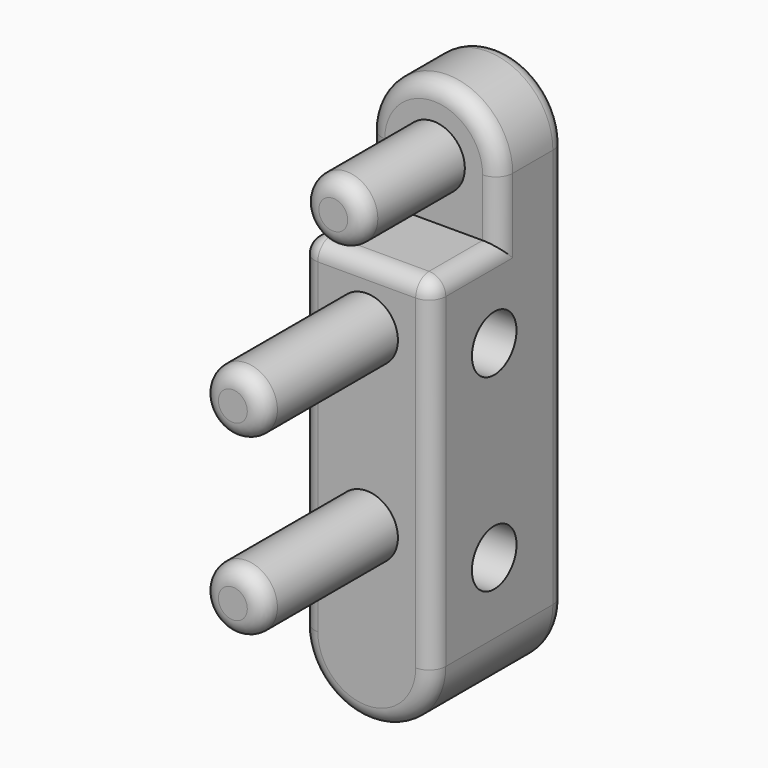
from build123d import *

# Parameters (mm, degrees)
F0_R     = 9.4597461698
F1_DEPTH = 101.6
F0_W     = 39.8592872384
F0_H     = 103.9333879682
F2_DEPTH = 50.8
F3_DEPTH = 25.4
F4_DEPTH = 63.5
F5_R     = 5.08
F6_R     = 5.08
F7_R     = 5.08
F8_R     = 8.4595796919
F9_DEPTH = 25.4
F12_R    = 5.08


# Not quite as in the source:
# - the program builds the solid bodies; features that only make, move or delete a surface that nothing else refers to are left out


with BuildPart() as f1:
    # F0 (on Front) → F1 (new body)
    with BuildSketch(Plane.XZ):
        with Locations((0, -35.6362370717)):
            Circle(F0_R)
    extrude(amount=F1_DEPTH)



with BuildPart() as f1b:
    # F0 (on Front) → F1, piece 2 (new body)
    with BuildSketch(Plane.XZ):
        with Locations((0, -88.4090361273)):
            Circle(F0_R)
    extrude(amount=F1_DEPTH)


with BuildPart() as f1_1:
    add(f1.part)

    add(f1b.part)  # F2 merges F1b
    # F0 (on Front) → F2 (join)
    with BuildSketch(Plane.XZ):
        with Locations((0, -69.4868988952)):
            Rectangle(F0_W, F0_H)
        with Locations((0, -88.4090361273)):
            Circle(F0_R, mode=Mode.SUBTRACT)
        with Locations((0, -35.6362370717)):
            Circle(F0_R, mode=Mode.SUBTRACT)
        with BuildLine():
            ThreePointArc((-19.9296436192, -121.4535928793), (0, -141.3832364985), (19.9296436192, -121.4535928793))
            Line((19.9296436192, -121.4535928793), (-19.9296436192, -121.4535928793))
        make_face()
    extrude(amount=F2_DEPTH)

    # F0 (on Front) → F3 (join)
    with BuildSketch(Plane.XZ):
        with BuildLine():
            Line((19.9296436192, -17.5202049111), (19.9296436192, 0))
            ThreePointArc((19.9296436192, 0), (0, 19.9296436192), (-19.9296436192, 0))
            Line((-19.9296436192, 0), (-19.9296436192, -17.5202049111))
            Line((-19.9296436192, -17.5202049111), (19.9296436192, -17.5202049111))
        make_face()
        Circle(F0_R, mode=Mode.SUBTRACT)
    extrude(amount=F3_DEPTH)

    # F0 (on Front) → F4 (join)
    with BuildSketch(Plane.XZ):
        Circle(F0_R)
    extrude(amount=F4_DEPTH)

    # F5
    f5_edges = [f1_1.edges().sort_by_distance(p)[0] for p in [
        (-19.929644, -50.8, -69.486899),
        (-19.929644, -38.1, -17.520205),
        (19.929644, -50.8, -69.486899),
        (0, -50.8, -17.520205),
        (19.929644, -38.1, -17.520205),
    ]]
    fillet(f5_edges, radius=F5_R)

    # F6
    f6_edges = [f1_1.edges().sort_by_distance(p)[0] for p in [
        (19.929644, 0, -60.726796),
        (0, 0, 19.929644),
        (-19.929644, 0, -60.726796),
        (0, 0, -141.383236),
    ]]
    fillet(f6_edges, radius=F6_R)

    # F7
    f7_edges = [f1_1.edges().sort_by_distance(p)[0] for p in [
        (-19.929644, -25.4, -8.760102),
        (-19.929644, -25.4, -20.060205),
        (0, -25.4, 19.929644),
        (19.929644, -15.24, 0),
    ]]
    fillet(f7_edges, radius=F7_R)

    # F8 (on Right) → F9 (cut, symmetric)
    with BuildSketch(Plane.YZ):
        with Locations((-27.3456163704, -42.5785966218)):
            Circle(F8_R)
        with Locations((-27.3456163704, -99.8373031616)):
            Circle(F8_R)
    extrude(amount=F9_DEPTH, both=True, mode=Mode.SUBTRACT)

    # F12
    f12_edges = [f1_1.edges().sort_by_distance(p)[0] for p in [
        (-9.459746, -101.6, -88.409036),
        (-9.459746, -101.6, -35.636237),
        (-9.459746, -63.5, 0),
    ]]
    fillet(f12_edges, radius=F12_R)


solid = f1_1.part
